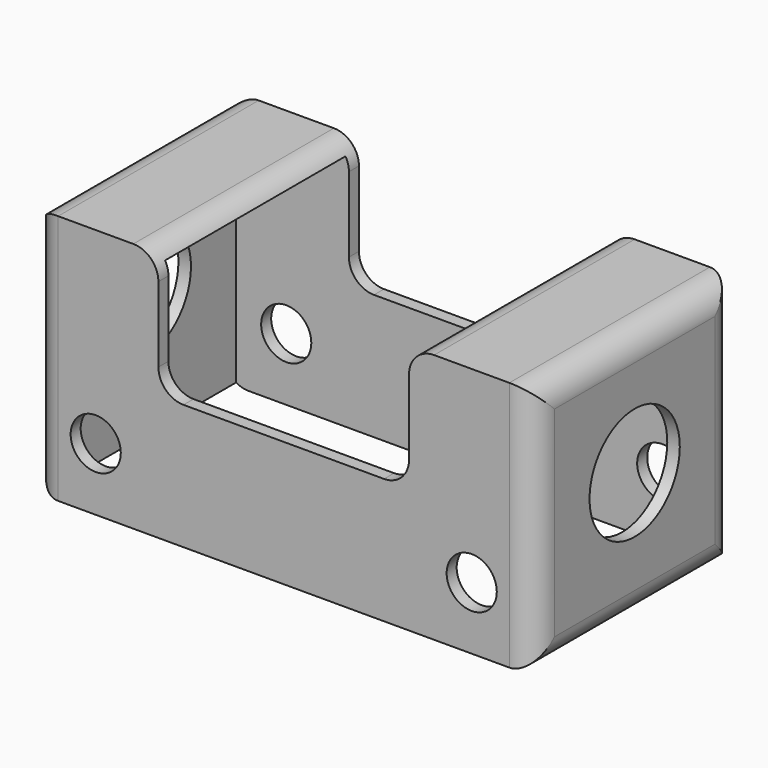
from build123d import *

# Parameters (mm, degrees)
F0_W        = 100
F0_H        = 50
F1_DEPTH    = 50
F2_T        = -2.5
F3_W        = 50
F3_H        = 70.2898527046
F4_DEPTH    = 25
F5_R        = 5
F6_DEPTH    = 50
F7_T1_DEPTH = 75
F7_T3_DEPTH = 75
F8_T1_DEPTH = 2.5
F8_T3_DEPTH = 2.5
F8_T5_DEPTH = 75
F9_T1_DEPTH = 75
F9_T3_DEPTH = 75
F10_R       = 11.25
F11_DEPTH   = 100


# Not quite as in the source:
# - a fillet or chamfer that OpenCascade refuses, or shapes differently, is made with other operations: its cross-section is extruded or revolved along the edge and cut away or added


with BuildPart() as f1:
    # F0 (on Top) → F1 (new body)
    with BuildSketch(Plane.XY):
        with Locations((50, 25)):
            Rectangle(F0_W, F0_H)
    extrude(amount=F1_DEPTH)

    # F2
    f2_openings = [f1.faces().sort_by_distance(p)[0] for p in [
        (50, 25, 0),
    ]]
    offset(amount=F2_T, openings=f2_openings)

    # F3 (on face) → F4 (cut)
    with BuildSketch(Plane.XY.offset(50)):
        with Locations((50, 24.9999999069)):
            Rectangle(F3_W, F3_H)
    extrude(amount=-F4_DEPTH, mode=Mode.SUBTRACT)

    # F5 (on face) → F6 (cut)
    with BuildSketch(Plane.XZ):
        with Locations((12.5, 12.5)):
            Circle(F5_R)
        with Locations((87.5, 12.5)):
            Circle(F5_R)
    extrude(amount=-F6_DEPTH, mode=Mode.SUBTRACT)

    # F7: fillet of radius 5 on 4 edges, made by hand

    # F7_s2 → F7_t1 (cut)
    with BuildSketch(Plane.XZ.offset(-62.5)):
        with BuildLine():
            ThreePointArc((0, 45), (1.4644660941, 48.5355339059), (5, 50))
            Line((5, 50), (0, 50))
            Line((0, 50), (0, 45))
        make_face()
        with BuildLine():
            ThreePointArc((0, 5), (1.4644660941, 1.4644660941), (5, 0))
            Line((5, 0), (0, 0))
            Line((0, 0), (0, 5))
        make_face()
    extrude(amount=F7_T1_DEPTH, mode=Mode.SUBTRACT)

    # F7_s4 → F7_t3 (cut)
    with BuildSketch(Plane.XY.offset(-12.5)):
        with BuildLine():
            ThreePointArc((0, 5), (1.4644660941, 1.4644660941), (5, 0))
            Line((5, 0), (0, 0))
            Line((0, 0), (0, 5))
        make_face()
        with BuildLine():
            ThreePointArc((0, 45), (1.4644660941, 48.5355339059), (5, 50))
            Line((5, 50), (0, 50))
            Line((0, 50), (0, 45))
        make_face()
    extrude(amount=F7_T3_DEPTH, mode=Mode.SUBTRACT)

    # F8: fillet of radius 5 on 6 edges, made by hand

    # F8_s2 → F8_t1 (join)
    with BuildSketch(Plane.XZ.offset(-2.5)):
        with BuildLine():
            ThreePointArc((25, 30), (26.4644660941, 26.4644660941), (30, 25))
            Line((30, 25), (25, 25))
            Line((25, 25), (25, 30))
        make_face()
        with BuildLine():
            ThreePointArc((75, 30), (73.5355339059, 26.4644660941), (70, 25))
            Line((70, 25), (75, 25))
            Line((75, 25), (75, 30))
        make_face()
    extrude(amount=F8_T1_DEPTH)

    # F8_s4 → F8_t3 (join)
    with BuildSketch(Plane.XZ.offset(-50)):
        with BuildLine():
            ThreePointArc((25, 30), (26.4644660941, 26.4644660941), (30, 25))
            Line((30, 25), (25, 25))
            Line((25, 25), (25, 30))
        make_face()
        with BuildLine():
            ThreePointArc((70, 25), (73.5355339059, 26.4644660941), (75, 30))
            Line((75, 30), (75, 25))
            Line((75, 25), (70, 25))
        make_face()
    extrude(amount=F8_T3_DEPTH)

    # F8_s6 → F8_t5 (cut)
    with BuildSketch(Plane.XZ.offset(-62.5)):
        with BuildLine():
            ThreePointArc((20, 50), (23.5355339059, 48.5355339059), (25, 45))
            Line((25, 45), (25, 50))
            Line((25, 50), (20, 50))
        make_face()
        with BuildLine():
            ThreePointArc((75, 45), (76.4644660941, 48.5355339059), (80, 50))
            Line((80, 50), (75, 50))
            Line((75, 50), (75, 45))
        make_face()
    extrude(amount=F8_T5_DEPTH, mode=Mode.SUBTRACT)

    # F9: fillet of radius 5 on 4 edges, made by hand

    # F9_s2 → F9_t1 (cut)
    with BuildSketch(Plane.XZ.offset(-62.5)):
        with BuildLine():
            ThreePointArc((100, 45), (98.5355339059, 48.5355339059), (95, 50))
            Line((95, 50), (100, 50))
            Line((100, 50), (100, 45))
        make_face()
        with BuildLine():
            ThreePointArc((95, 0), (98.5355339059, 1.4644660941), (100, 5))
            Line((100, 5), (100, 0))
            Line((100, 0), (95, 0))
        make_face()
    extrude(amount=F9_T1_DEPTH, mode=Mode.SUBTRACT)

    # F9_s4 → F9_t3 (cut)
    with BuildSketch(Plane.XY.offset(-12.5)):
        with BuildLine():
            ThreePointArc((95, 0), (98.5355339059, 1.4644660941), (100, 5))
            Line((100, 5), (100, 0))
            Line((100, 0), (95, 0))
        make_face()
        with BuildLine():
            ThreePointArc((95, 50), (98.5355339059, 48.5355339059), (100, 45))
            Line((100, 45), (100, 50))
            Line((100, 50), (95, 50))
        make_face()
    extrude(amount=F9_T3_DEPTH, mode=Mode.SUBTRACT)

    # F10 (on face) → F11 (cut)
    with BuildSketch(Plane.YZ.offset(100)):
        with Locations((25, 25.6698729811)):
            Circle(F10_R)
    extrude(amount=-F11_DEPTH, mode=Mode.SUBTRACT)


solid = f1.part
